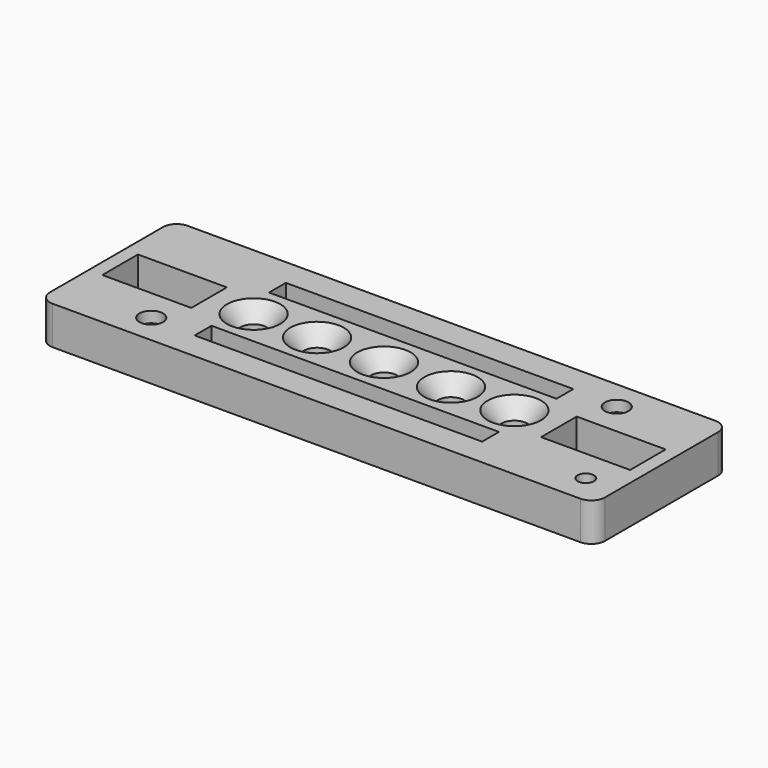
from build123d import *

# Parameters (mm, degrees)
F0_W           = 81.1
F0_H           = 24.65
F1_DEPTH       = 5.6
F3_D           = 3.45
F4_D           = 2.39
F6_D           = 3.7973
F6_CSINK_D     = 7.7978
F6_CSINK_ANGLE = 82
F7_R           = 1.725
F7_R_2         = 1.195
F8_DEPTH       = 3.9998
F7_W           = 42
F7_H           = 3.075
F7_W_2         = 13
F7_H_2         = 6.5
F9_DEPTH       = 5.6
F10_R          = 2


# Not quite as in the source:
# - a feature names something its author has since deleted; it is built from what else it names


with BuildPart() as f1:
    # F0 (on Top) → F1 (new body)
    with BuildSketch(Plane.XY):
        Rectangle(F0_W, F0_H)
    extrude(amount=F1_DEPTH)

    # F3 (through all)
    with Locations(Plane.XY.offset(5.6)):
        with Locations((-27.6, -8), (27.6, 8)):
            Hole(F3_D / 2)

    # F4 (through all)
    with Locations(Plane.XY.offset(5.6)):
        with Locations((35.88, -8)):
            Hole(F4_D / 2)

    # F6 (through all)
    with Locations(Plane.XY.offset(5.6)):
        with Locations((-19.05, 0), (-9.779, 0), (0, 0), (9.779, 0), (19.05, 0)):
            CounterSinkHole(F6_D / 2, F6_CSINK_D / 2, counter_sink_angle=F6_CSINK_ANGLE)

    # F7 (on face) → F8 (cut, through all)
    with BuildSketch(Plane(origin=(0, 0, 0), x_dir=(1, 0, 0), z_dir=(0, 0, -1))):
        Polygon((-38.55, 10.325), (-38.55, 5.25), (-23.55, 5.25), (-23, 5.25), (-23, 10.325), align=None)
        with Locations((-27.6, 8)):
            Circle(F7_R, mode=Mode.SUBTRACT)
        Polygon((-23.55, -5.25), (-38.55, -5.25), (-38.55, -10.325), (-23, -10.325), (-23, -5.25), align=None)
        Polygon((38.55, -10.325), (38.55, -5.25), (23.55, -5.25), (23, -5.25), (23, -10.325), align=None)
        with Locations((27.6, -8)):
            Circle(F7_R, mode=Mode.SUBTRACT)
        Polygon((23.55, 5.25), (38.55, 5.25), (38.55, 10.325), (23, 10.325), (23, 5.25), align=None)
        with Locations((35.88, 8)):
            Circle(F7_R_2, mode=Mode.SUBTRACT)
    extrude(amount=-F8_DEPTH, mode=Mode.SUBTRACT)

    # F7 (on face) → F9 (cut, through all)
    with BuildSketch(Plane(origin=(0, 0, 0), x_dir=(1, 0, 0), z_dir=(0, 0, -1))):
        with Locations((0, -6.7875)):
            Rectangle(F7_W, F7_H)
        with Locations((-32.05, 0)):
            Rectangle(F7_W_2, F7_H_2)
        with Locations((32.05, 0)):
            Rectangle(F7_W_2, F7_H_2)
        with Locations((0, 6.7875)):
            Rectangle(F7_W, F7_H)
    extrude(amount=-F9_DEPTH, mode=Mode.SUBTRACT)

    # F10
    f10_edges = [f1.edges().sort_by_distance(p)[0] for p in [
        (40.55, 12.325, 2.8),
        (-40.55, 12.325, 2.8),
        (-40.55, -12.325, 2.8),
        (40.55, -12.325, 2.8),
    ]]
    fillet(f10_edges, radius=F10_R)


solid = f1.part
